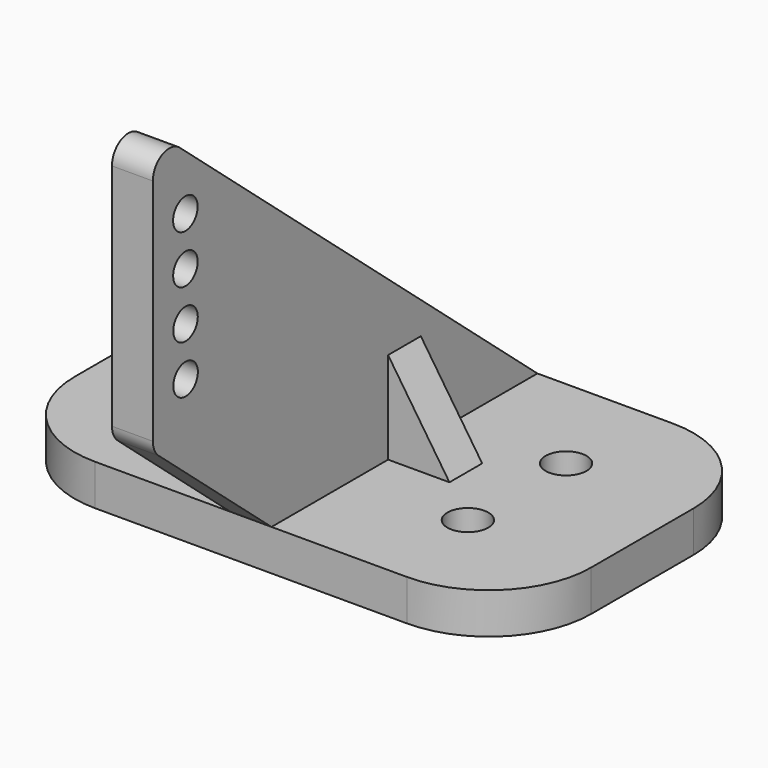
from build123d import *

# Parameters (mm, degrees)
F0_R     = 1
F0_W     = 2
F0_H     = 2
F0_H_2   = 7.125
F0_W_2   = 3
F1_DEPTH = 2
F2_R     = 0.75
F3_DEPTH = 1
F5_DEPTH = 1


# Not quite as in the source:
# - ends of sketch curves that miss each other by under 0.0002 mm in the source are joined


with BuildPart() as f1:
    # F0 (on Top) → F1 (new body)
    with BuildSketch(Plane.XY):
        with BuildLine():
            Line((6.5, -8.125), (7.625, -8.125))
            ThreePointArc((7.625, -8.125), (11.1605339059, -6.6605339059), (12.625, -3.125))
            Line((12.625, -3.125), (12.625, -3))
            Line((12.625, -3), (12.625, -1))
            Line((12.625, -1), (12.625, 1))
            Line((12.625, 1), (12.625, 3))
            Line((12.625, 3), (12.625, 3.125))
            ThreePointArc((12.625, 3.125), (11.1605339059, 6.6605339059), (7.625, 8.125))
            Line((7.625, 8.125), (6.5, 8.125))
            Line((6.5, 8.125), (1, 8.125))
            Line((1, 8.125), (1, 1))
            Line((1, 1), (4, 1))
            Line((4, 1), (4, -1))
            Line((4, -1), (1, -1))
            Line((1, -1), (1, -8.125))
            Line((1, -8.125), (6.5, -8.125))
        make_face()
        with Locations((6.5, -3)):
            Circle(F0_R, mode=Mode.SUBTRACT)
        with Locations((6.5, 3)):
            Circle(F0_R, mode=Mode.SUBTRACT)
        with BuildLine():
            Line((-6.5, -8.125), (-1, -8.125))
            Line((-1, -8.125), (-1, -1))
            Line((-1, -1), (-4, -1))
            Line((-4, -1), (-4, 1))
            Line((-4, 1), (-1, 1))
            Line((-1, 1), (-1, 8.125))
            Line((-1, 8.125), (-6.5, 8.125))
            Line((-6.5, 8.125), (-7.625, 8.125))
            ThreePointArc((-7.625, 8.125), (-11.1605339059, 6.6605339059), (-12.625, 3.125))
            Line((-12.625, 3.125), (-12.625, 3))
            Line((-12.625, 3), (-12.625, 1))
            Line((-12.625, 1), (-12.625, -1))
            Line((-12.625, -1), (-12.625, -3))
            Line((-12.625, -3), (-12.625, -3.125))
            ThreePointArc((-12.625, -3.125), (-11.1605339059, -6.6605339059), (-7.625, -8.125))
            Line((-7.625, -8.125), (-6.5, -8.125))
        make_face()
        with Locations((-6.5, -3)):
            Circle(F0_R, mode=Mode.SUBTRACT)
        with Locations((-6.5, 3)):
            Circle(F0_R, mode=Mode.SUBTRACT)
        Rectangle(F0_W, F0_H)
        with Locations((0, 4.5625)):
            Rectangle(F0_W, F0_H_2)
        with Locations((0, -4.5625)):
            Rectangle(F0_W, F0_H_2)
        with Locations((2.5, 0)):
            Rectangle(F0_W_2, F0_H)
        with Locations((-2.5, 0)):
            Rectangle(F0_W_2, F0_H)
    extrude(amount=-F1_DEPTH)


with BuildPart() as f3:
    # F2 (on Right) → F3 (new body, symmetric)
    with BuildSketch(Plane.YZ):
        with BuildLine():
            Line((-8.1246402115, 0), (0, 0))
            Line((0, 0), (8.1249158829, 0))
            Line((8.1249158829, 0), (-13.7268813705, 18.5973458472))
            ThreePointArc((-13.7268813705, 18.5973458472), (-14.7944528403, 18.7435835859), (-15.375, 17.8358064575))
            Line((-15.375, 17.8358064575), (-15.375, 6.6325848519))
            ThreePointArc((-15.375, 6.6325848519), (-15.2827771284, 6.2131320116), (-15.0231186295, 5.8710454622))
            Line((-15.0231186295, 5.8710454622), (-8.1246402115, 0))
        make_face()
        with Locations((-13.375, 8.5)):
            Circle(F2_R, mode=Mode.SUBTRACT)
        with Locations((-13.379498098, 10.8749957404)):
            Circle(F2_R, mode=Mode.SUBTRACT)
        with Locations((-13.383996196, 13.2499914809)):
            Circle(F2_R, mode=Mode.SUBTRACT)
        with Locations((-13.388494294, 15.6249872213)):
            Circle(F2_R, mode=Mode.SUBTRACT)
    extrude(amount=F3_DEPTH, both=True)


with BuildPart() as f5:
    # F4 (on Front) → F5 (new body, symmetric)
    with BuildSketch(Plane.XZ):
        Polygon((-4, 0), (-1, 0), (-1, 4.5), align=None)
    extrude(amount=F5_DEPTH, both=True)


with BuildPart() as f5b:
    # F4 (on Front) → F5, piece 2 (new body, symmetric)
    with BuildSketch(Plane.XZ):
        Polygon((1, 4.5), (1, 0), (4, 0), align=None)
    extrude(amount=F5_DEPTH, both=True)


solid = Compound([f1.part, f3.part, f5.part, f5b.part])
